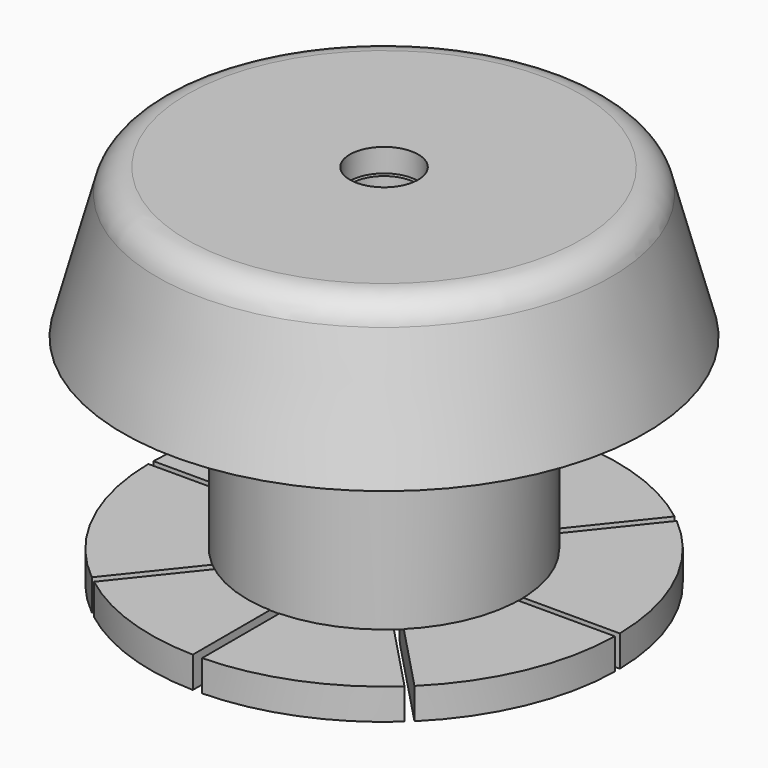
from build123d import *

# Parameters (mm, degrees)
F2_SIZE2       = 4
F2_SIZE        = 2
F3_W           = 34.7070610151
F3_H           = 15.6652256846
F4_DEPTH       = 0.2
F4_DEPTH_BACK  = 0.2
F5_R           = 1
F8_R           = 2
F10_D          = 1.5
F10_DEPTH      = 14.9996666074
F11_D          = 1.5
F12_W          = 46.682305634
F12_H          = 21.989823319
F13_DEPTH      = 0.3
F13_DEPTH_BACK = 0.3
F14_R          = 1
F15_R          = 0.732099207
F16_DEPTH      = 25
F16_DEPTH_BACK = 25
F18_DEPTH      = 10


with BuildPart() as f1:
    # F0 (on Front) → F1 (revolve)
    with BuildSketch(Plane.XZ):
        with BuildLine():
            Line((-15, 0), (-4.5, 0))
            Line((-4.5, 0), (-4.5, 5))
            ThreePointArc((-4.5, 5), (-5.6803746274, 8.9711640828), (-3.8599889164, 12.6926724191))
            Line((-3.8599889164, 12.6926724191), (-3.8599889164, 13.85303602))
            Line((-3.8599889164, 13.85303602), (-3.75, 17))
            Line((-3.75, 17), (-3.75, 18.085423857))
            Line((-3.75, 18.085423857), (-2.1, 18.6220947653))
            Line((-2.1, 18.6220947653), (-2.1, 22))
            Line((-2.1, 22), (-6.2739714049, 22))
            Line((-6.2739714049, 22), (-6.2739714049, 17))
            Line((-6.2739714049, 17), (-7.5, 17))
            Line((-7.5, 17), (-7.5, 2))
            Line((-7.5, 2), (-15, 2))
            Line((-15, 2), (-15, 0))
        make_face()
    revolve(axis=Axis((0, 0, -0.9101470151), (0, 0, -1)))

    # F2
    f2_edges = [f1.edges().sort_by_distance(p)[0] for p in [
        (4.5, 0, 0),
    ]]
    chamfer(f2_edges, length=F2_SIZE, length2=F2_SIZE2)

    # F3 (on Front) → F4 (cut, two sides)
    with BuildSketch(Plane.XZ) as f4_sk:
        with Locations((0.8775419556, 3.662395291)):
            Rectangle(F3_W, F3_H)
    extrude(amount=F4_DEPTH, mode=Mode.SUBTRACT)
    extrude(f4_sk.sketch, amount=-F4_DEPTH_BACK, mode=Mode.SUBTRACT)

    # F5
    f5_edges = [f1.edges().sort_by_distance(p)[0] for p in [
        (7.5, 0, 17),
        (6.273971, 0, 22),
    ]]
    fillet(f5_edges, radius=F5_R)

    # F10 (through all, one way)
    with BuildSketch(Plane.YZ):
        with Locations((0, 11.4683825523)):
            Circle(F10_D / 2)
    extrude(amount=-F10_DEPTH, mode=Mode.SUBTRACT)

    # F11 (through all)
    with Locations(Plane(origin=(0, 0, 0), x_dir=(0, 1, 0), z_dir=(-1, 0, 0))):
        with Locations((0, -11.4683825523)):
            Hole(F11_D / 2)

    # F12 (on Right) → F13 (cut, two sides)
    with BuildSketch(Plane.YZ) as f13_sk:
        with Locations((-1.1946484447, 0.5094152875)):
            Rectangle(F12_W, F12_H)
    extrude(amount=F13_DEPTH, mode=Mode.SUBTRACT)
    extrude(f13_sk.sketch, amount=-F13_DEPTH_BACK, mode=Mode.SUBTRACT)

    # F15 (on Front) → F16 (cut, two sides)
    with BuildSketch(Plane.XZ) as f16_sk:
        with Locations((0, 11.4638349041)):
            Circle(F15_R)
    extrude(amount=-F16_DEPTH, mode=Mode.SUBTRACT)
    extrude(f16_sk.sketch, amount=F16_DEPTH_BACK, mode=Mode.SUBTRACT)

    # F17 (on face) → F18 (cut)
    with BuildSketch(Plane(origin=(0, 0, 0), x_dir=(1, 0, 0), z_dir=(0, 0, -1))):
        with BuildLine():
            ThreePointArc((10.5139905017, 10.6984112713), (10.3342231343, 10.872158581), (10.1515849457, 11.0428856324))
            Line((10.1515849457, 11.0428856324), (4.2858445251, 4.8868739196))
            ThreePointArc((4.2858445251, 4.8868739196), (4.4706307589, 4.7184171729), (4.6488011335, 4.5429778803))
            Line((4.6488011335, 4.5429778803), (10.5139905017, 10.6984112713))
        make_face()
        with BuildLine():
            ThreePointArc((4.6488011335, 4.5429778803), (4.4706307589, 4.7184171729), (4.2858445251, 4.8868739196))
            Line((4.2858445251, 4.8868739196), (0.036769962, 0.4275301875))
            Line((0.036769962, 0.4275301875), (0.3515986607, 0.0331245868))
            Line((0.3515986607, 0.0331245868), (4.6488011335, 4.5429778803))
        make_face()
        with BuildLine():
            Line((-0.3092622619, 0.0643742565), (0.036769962, 0.4275301875))
            Line((0.036769962, 0.4275301875), (-3.8199505928, 5.2590852312))
            ThreePointArc((-3.8199505928, 5.2590852312), (-4.0184659824, 5.1090049078), (-4.2110908751, 4.9514355132))
            Line((-4.2110908751, 4.9514355132), (-0.3092622619, 0.0643742565))
        make_face()
        Polygon((0.0056016096, -0.3299944307), (-0.3092622619, 0.0643742565), (-23.7269770598, -24.5121866283), (-23.3649924477, -24.8571027639), align=None)
        Polygon((10.0267531176, -12.0875464992), (0.3515986607, 0.0331245868), (0.0056016096, -0.3299944307), (9.681836982, -12.4495311113), align=None)
        with BuildLine():
            ThreePointArc((-4.2110908751, 4.9514355132), (-4.0184659824, 5.1090049078), (-3.8199505928, 5.2590852312))
            Line((-3.8199505928, 5.2590852312), (-9.1250853215, 11.9051592965))
            ThreePointArc((-9.1250853215, 11.9051592965), (-9.3216393624, 11.7518951492), (-9.5156196617, 11.5953862572))
            Line((-9.5156196617, 11.5953862572), (-4.2110908751, 4.9514355132))
        make_face()
        with BuildLine():
            ThreePointArc((-9.5156196617, 11.5953862572), (-9.3216393624, 11.7518951492), (-9.1250853215, 11.9051592965))
            Line((-9.1250853215, 11.9051592965), (-11.4102009684, 14.7678665817))
            Line((-11.4102009684, 14.7678665817), (-11.7787780998, 14.4300043343))
            Line((-11.7787780998, 14.4300043343), (-9.5156196617, 11.5953862572))
        make_face()
    extrude(amount=-F18_DEPTH, mode=Mode.SUBTRACT)


with BuildPart() as f7:
    # F6 (on Front) → F7 (revolve)
    with BuildSketch(Plane.XZ):
        Polygon((-14.2, 23.6), (-16.8, 14), (-8.8, 14), (-8.8, 17.4), (-8.7994168971, 17.4), (-7.6, 17.4), (-6.5739714049, 17.4), (-6.5739714049, 22.1), (-2.2, 22.1), (-2.2, 23.6), align=None)
        Polygon((-7.6, 17.4), (-8.7994168971, 17.4), (-8.7994168971, 1.9800447152), (-7.6, 2.0174493548), align=None)
    revolve(axis=Axis((0, 0, -0.9101470151), (0, 0, -1)))

    # F8
    f8_edges = [f7.edges().sort_by_distance(p)[0] for p in [
        (14.2, 0, 23.6),
    ]]
    fillet(f8_edges, radius=F8_R)

    # F14
    f14_edges = [f7.edges().sort_by_distance(p)[0] for p in [
        (7.6, 0, 2.017449),
    ]]
    fillet(f14_edges, radius=F14_R)


solid = Compound([f1.part, f7.part])
